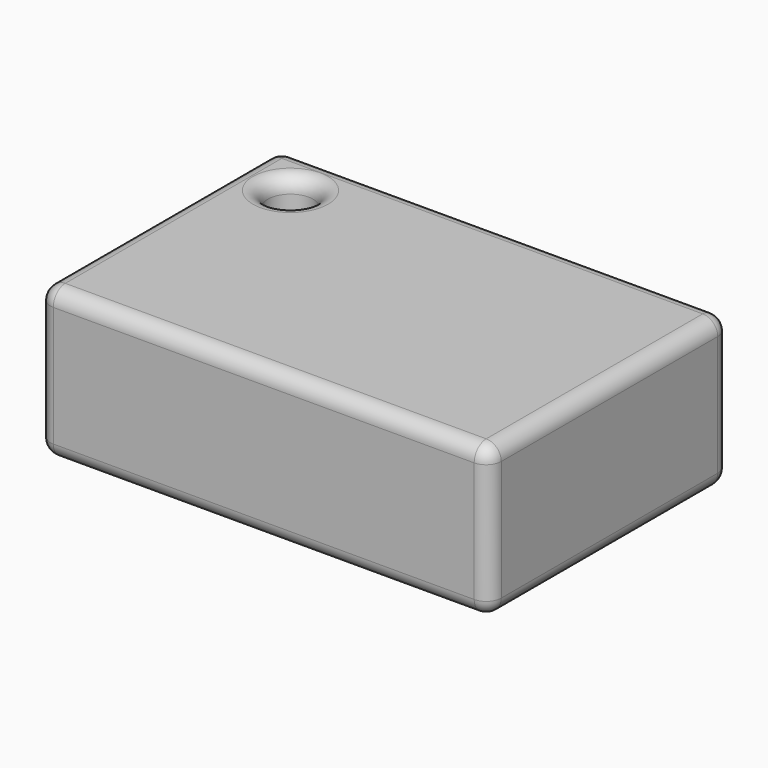
from build123d import *

# Parameters (mm, degrees)
F0_W        = 300
F0_H        = 200
F0_R        = 15
F1_DEPTH    = 100
F2_R        = 10
F3_T1_DEPTH = 115
F3_S5_W     = 10
F3_S5_H     = 10
F3_T6_DEPTH = 10
F4_R        = 10


# Not quite as in the source:
# - a fillet or chamfer that OpenCascade refuses, or shapes differently, is made with other operations: its cross-section is extruded or revolved along the edge and cut away or added


with BuildPart() as f1:
    # F0 (on Top) → F1 (new body)
    with BuildSketch(Plane.XY):
        with Locations((-14.5989330485, 4.2332556737)):
            Rectangle(F0_W, F0_H)
        with Locations((-128.6004347833, 68.9842231594)):
            Circle(F0_R, mode=Mode.SUBTRACT)
    extrude(amount=F1_DEPTH)

    # F2
    f2_edges = [f1.edges().sort_by_distance(p)[0] for p in [
        (-164.598933, 104.233256, 50),
        (-14.598933, 104.233256, 100),
        (135.401067, 104.233256, 50),
        (135.401067, 4.233256, 100),
        (-164.598933, 4.233256, 100),
        (-143.600435, 68.984223, 100),
        (135.401067, -95.766744, 50),
        (-14.598933, -95.766744, 100),
    ]]
    fillet(f2_edges, radius=F2_R)

    # F3: fillet of radius 10 on 3 edges, made by hand

    # F3_s2 → F3_t1 (cut)
    with BuildSketch(Plane.XY.offset(-25)):
        with BuildLine():
            ThreePointArc((-154.5989330485, -95.7667443263), (-161.6700008604, -92.8378121382), (-164.5989330485, -85.7667443263))
            Line((-164.5989330485, -85.7667443263), (-164.5989330485, -95.7667443263))
            Line((-164.5989330485, -95.7667443263), (-154.5989330485, -95.7667443263))
        make_face()
    extrude(amount=F3_T1_DEPTH, mode=Mode.SUBTRACT)


with BuildPart() as f3_tool4:
    # F3_s5 → F3_t6 (new body)
    with BuildSketch(Plane.XZ.offset(85.7667443263)):
        with Locations((-159.5989330485, 95)):
            Rectangle(F3_S5_W, F3_S5_H)
    extrude(amount=F3_T6_DEPTH)

    # F3_s7 → F3_t8 (revolve, cut)
    with BuildSketch(Plane(origin=(-154.5989330485, -85.7667443263, 90), x_dir=(0.7071067812, 0, -0.7071067812), z_dir=(-0.7071067812, 0, -0.7071067812))):
        with BuildLine():
            ThreePointArc((0, -10), (10, 0), (0, 10))
            Line((0, 10), (0, -10))
        make_face()
    revolve(axis=Axis((-154.5989330485, -85.7667443263, 90), (0, -1, 0)), mode=Mode.SUBTRACT)


with BuildPart() as f1_1:
    add(f1.part)

    # F3_t3: cut F3_tool4
    add(f3_tool4.part, mode=Mode.SUBTRACT)

    # F4
    f4_edges = [f1_1.edges().sort_by_distance(p)[0] for p in [
        (125.401067, 104.233256, 45),
        (135.401067, 94.233256, 45),
        (-154.598933, 104.233256, 45),
        (-161.670001, 101.304323, 0),
        (-164.598933, 94.233256, 45),
        (-161.670001, 101.304323, 90),
    ]]
    fillet(f4_edges, radius=F4_R)


solid = f1_1.part
